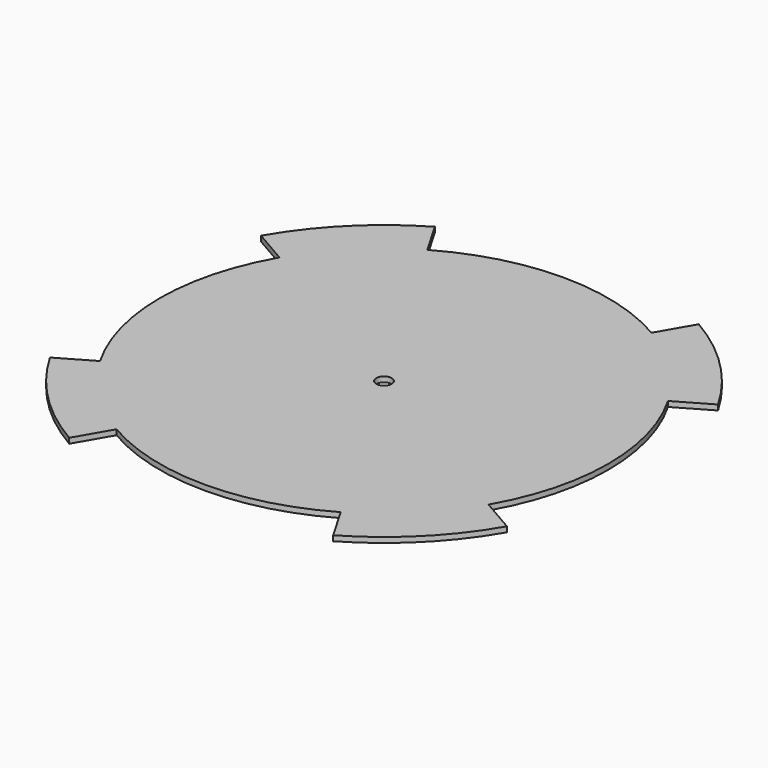
from build123d import *

# Parameters (mm, degrees)
F0_R            = 85
F1_DEPTH        = 2
F3_DEPTH        = 2
F3_COPIES_COUNT = 4
F4_R            = 2.95
F5_DEPTH        = 25


# Not quite as in the source:
# - a pattern or mirror of a feature is missing from the dataset's text; its kind, count and spacing are read off the source's solid
# - a feature names something its author has since deleted; it is built from what else it names


with BuildPart() as f1:
    # F0 (on Top) → F1 (new body)
    with BuildSketch(Plane.XY):
        Circle(F0_R)
    extrude(amount=F1_DEPTH)

    # F2 (on face) → F3 (join)
    with BuildSketch(Plane.XY.offset(2)):
        with BuildLine():
            ThreePointArc((-42.5, -73.6121593217), (-60.1040764009, -60.1040764009), (-73.6121593217, -42.5))
            Line((-73.6121593217, -42.5), (-86.6025403784, -50))
            ThreePointArc((-86.6025403784, -50), (-70.7106781187, -70.7106781187), (-50, -86.6025403784))
            Line((-50, -86.6025403784), (-42.5, -73.6121593217))
        make_face()
    f3 = extrude(amount=-F3_DEPTH)

    # F3_copies: F3 ×4 about axis
    f3_copies_axis = Axis((0, 0, 0), (0, 0, 1))
    for i in range(1, F3_COPIES_COUNT):
        add(f3.rotate(f3_copies_axis, i * 360 / F3_COPIES_COUNT))

    # F4 (on face) → F5 (cut)
    with BuildSketch(Plane(origin=(0, 0, 0), x_dir=(1, 0, 0), z_dir=(0, 0, -1))):
        Circle(F4_R)
    extrude(amount=-F5_DEPTH, mode=Mode.SUBTRACT)


solid = f1.part
